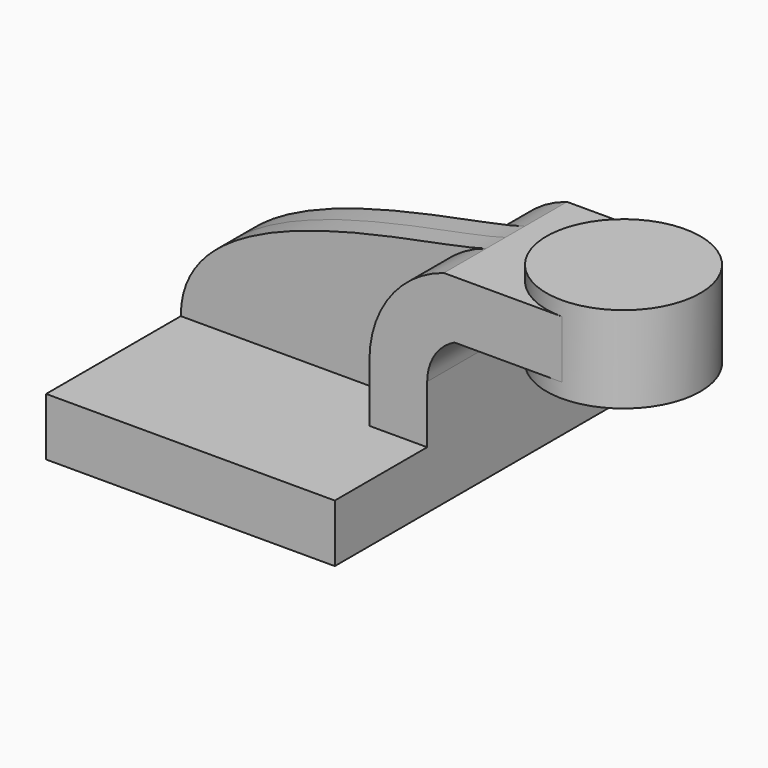
from build123d import *

# Parameters (mm, degrees)
F1_DEPTH = 63.5
F0_W     = 25.4
F0_H     = 19.05
F2_DEPTH = 25.4
F3_DEPTH = 7.9375


# Not quite as in the source:
# - ends of sketch curves that miss each other by under 0.0002 mm in the source are joined


with BuildPart() as f1:
    # F0 (on Front) → F1 (new body, symmetric)
    with BuildSketch(Plane.XZ):
        Polygon((-47.625, -9.525), (47.625, -9.525), (47.625, 9.525), (28.575, 9.525), (-47.625, 9.525), align=None)
    extrude(amount=F1_DEPTH, both=True)

    # F0 (on Front) → F2 (join, symmetric)
    with BuildSketch(Plane.XZ):
        with BuildLine():
            Line((28.575, 9.525), (47.625, 9.525))
            Line((47.625, 9.525), (47.625, 28.575))
            ThreePointArc((47.625, 28.575), (50.0566106583, 37.0183943417), (56.6065317176, 42.8752))
            Line((56.6065317176, 42.8752), (66.675, 42.8752))
            Line((66.675, 42.8752), (66.675, 61.9252))
            Line((66.675, 61.9252), (53.1308252517, 61.9252))
            ThreePointArc((53.1308252517, 61.9252), (35.3761751083, 49.2826338209), (28.575, 28.575))
            Line((28.575, 28.575), (28.575, 9.525))
        make_face()
        with Locations((79.375, 52.4002)):
            Rectangle(F0_W, F0_H)
    extrude(amount=F2_DEPTH, both=True)

    # F0 (on Front) → F3 (join, symmetric)
    with BuildSketch(Plane.XZ):
        with BuildLine():
            add(Edge.make_bspline(
                [(-47.625, 9.525), (-47.7196462452, 49.2661185562), (32.2834988688, 55.4433926855), (53.1308252517, 61.9252)],
                knots=[0, 0, 0, 0, 113.5672368344, 113.5672368344, 113.5672368344, 113.5672368344], degree=3))
            Line((-47.625, 9.525), (28.575, 9.525))
            Line((28.575, 9.525), (28.575, 28.575))
            ThreePointArc((28.575, 28.575), (35.3761751083, 49.2826338209), (53.1308252517, 61.9252))
        make_face()
    extrude(amount=F3_DEPTH, both=True)

    # F0 (on Front) → F4 (revolve)
    with BuildSketch(Plane.XZ):
        Polygon((92.075, 66.675), (92.075, 61.9252), (92.075, 42.8752), (92.075, 38.1), (117.475, 38.1), (117.475, 66.675), align=None)
    revolve(axis=Axis((92.075, 0, 52.3875), (0, 0, 1)))


solid = f1.part
